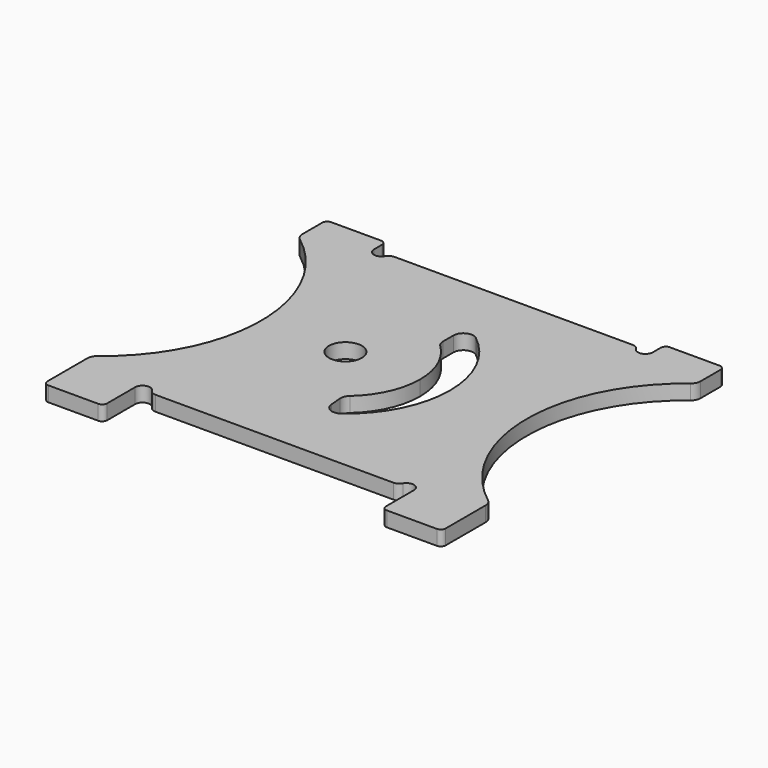
from build123d import *

# Parameters (mm, degrees)
F0_R     = 1.65
F1_DEPTH = 1.5
F2_R     = 1


# Not quite as in the source:
# - ends of sketch curves that miss each other by under 0.0002 mm in the source are joined


with BuildPart() as f1:
    # F0 (on Top) → F1 (new body)
    with BuildSketch(Plane.XY):
        with BuildLine():
            ThreePointArc((19.6082164698, -11.4503983868), (13.339608, 1.2499996959), (19.608215987, 13.9503980169))
            ThreePointArc((19.608215987, 13.9503980169), (19.8967236619, 14.3015730303), (20.000004, 14.744172))
            Line((20.000004, 14.744172), (20.000004, 17.25))
            ThreePointArc((20.000004, 17.25), (19.8535573906, 17.6035533906), (19.500004, 17.75))
            Line((19.500004, 17.75), (14.500004, 17.75))
            ThreePointArc((14.500004, 17.75), (14.1464506094, 17.6035533906), (14.000004, 17.25))
            Line((14.000004, 17.25), (14.000004, 16.25))
            ThreePointArc((14.000004, 16.25), (13.4441182966, 15.5255556337), (12.6004849604, 15.8749999771))
            ThreePointArc((12.6004849604, 15.8749999771), (12.3259659886, 16.1495190594), (11.950966, 16.25))
            Line((11.950966, 16.25), (-11.950958, 16.25))
            ThreePointArc((-11.950958, 16.25), (-12.3259579886, 16.1495190594), (-12.6004770396, 15.8750000229))
            ThreePointArc((-12.6004770396, 15.8750000229), (-13.4441102966, 15.5255556337), (-13.999996, 16.25))
            Line((-13.999996, 16.25), (-13.999996, 17.25))
            ThreePointArc((-13.999996, 17.25), (-14.1464426094, 17.6035533906), (-14.499996, 17.75))
            Line((-14.499996, 17.75), (-19.499996, 17.75))
            ThreePointArc((-19.499996, 17.75), (-19.8535493906, 17.6035533906), (-19.999996, 17.25))
            Line((-19.999996, 17.25), (-19.999996, 14.744172))
            ThreePointArc((-19.999996, 14.744172), (-19.8967156619, 14.3015730303), (-19.6082083041, 13.9503976031))
            ThreePointArc((-19.6082083041, 13.9503976031), (-13.3396, 1.2499996959), (-19.6082084698, -11.4503983868))
            ThreePointArc((-19.6082084698, -11.4503983868), (-19.8967227718, -11.8015703601), (-20.000004, -12.244173))
            Line((-20.000004, -12.244173), (-19.999996, -17.25))
            ThreePointArc((-19.999996, -17.25), (-19.8535493906, -17.6035533906), (-19.499996, -17.75))
            Line((-19.499996, -17.75), (-14.499996, -17.75))
            ThreePointArc((-14.499996, -17.75), (-14.1464426094, -17.6035533906), (-13.999996, -17.25))
            Line((-13.999996, -17.25), (-13.999996, -13.75))
            ThreePointArc((-13.999996, -13.75), (-13.4441102966, -13.0255556337), (-12.6004769604, -13.3749999771))
            ThreePointArc((-12.6004769604, -13.3749999771), (-12.3259579886, -13.6495190594), (-11.950958, -13.75))
            Line((-11.950958, -13.75), (11.950966, -13.75))
            ThreePointArc((11.950966, -13.75), (12.3259659886, -13.6495190594), (12.6004850396, -13.3750000229))
            ThreePointArc((12.6004850396, -13.3750000229), (13.4441182966, -13.0255556337), (14.000004, -13.75))
            Line((14.000004, -13.75), (14.000004, -17.25))
            ThreePointArc((14.000004, -17.25), (14.1464506094, -17.6035533906), (14.500004, -17.75))
            Line((14.500004, -17.75), (19.500004, -17.75))
            ThreePointArc((19.500004, -17.75), (19.8535573906, -17.6035533906), (20.000004, -17.25))
            Line((20.000004, -17.25), (20.000004, -12.244173))
            ThreePointArc((20.000004, -12.244173), (19.8967236619, -11.8015740303), (19.6082164698, -11.4503983868))
        make_face()
        with Locations((-4.8728769961, 1.25)):
            Circle(F0_R, mode=Mode.SUBTRACT)
        with BuildLine():
            ThreePointArc((-0.3045548123, -4.6981452929), (1.8543964627, -2.0656887385), (2.6271230039, 1.25))
            ThreePointArc((2.6271230039, 1.25), (1.938751938, 4.3887435806), (0, 6.9513217574))
            Line((0, 6.9513217574), (0, 10.550810168))
            ThreePointArc((0, 10.550810168), (4.1108641083, 6.6852916914), (5.6271230039, 1.25))
            ThreePointArc((5.6271230039, 1.25), (4.1108641083, -4.1852916914), (0, -8.050810168))
            Line((0, -8.050810168), (-0.3045548123, -4.6981452929))
        make_face(mode=Mode.SUBTRACT)
    extrude(amount=F1_DEPTH)

    # F2
    f2_edges = [f1.edges().sort_by_distance(p)[0] for p in [
        (0, 10.55081, 0.75),
        (-0.304555, -4.698145, 0.75),
        (0, -8.05081, 0.75),
        (0, 6.951322, 0.75),
    ]]
    fillet(f2_edges, radius=F2_R)


solid = f1.part
